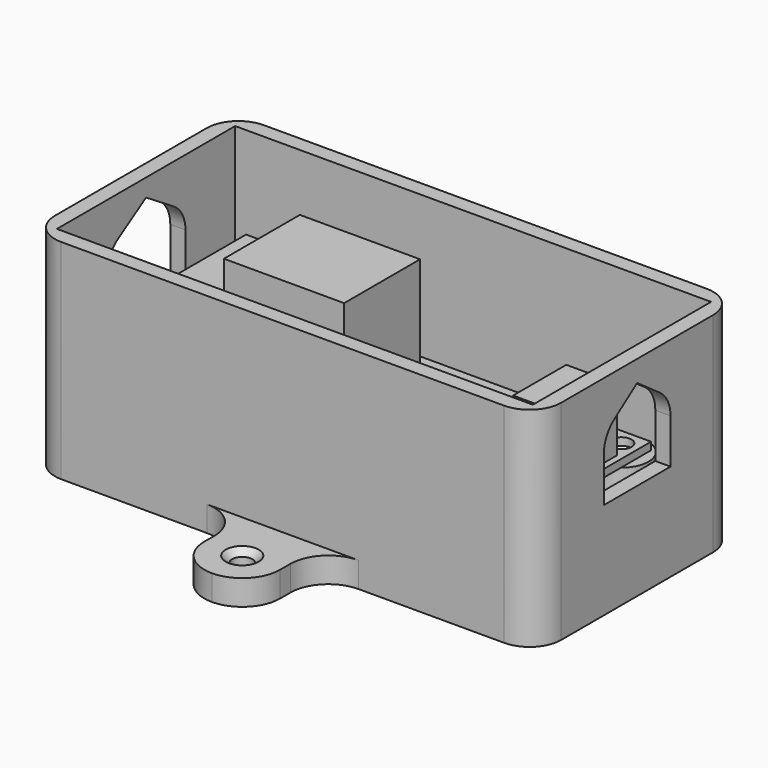
from build123d import *

# Parameters (mm, degrees)
F1_W          = 67.6
F1_H          = 21
F1_R          = 1.6
F2_DEPTH      = 1.2
F3_W          = 80
F3_H          = 40
F3_W_2        = 52
F3_H_2        = 28
F4_DEPTH      = 3
F5_R          = 4.25
F5_R_2        = 1.25
F6_DEPTH      = 14
F7_W          = 8
F7_H          = 15
F7_H_2        = 10.5
F8_DEPTH      = 10
F9_W          = 19
F9_H          = 15
F10_DEPTH     = 15.5
F11_W         = 80
F11_H         = 40
F11_W_2       = 75.2
F11_H_2       = 35.2
F12_DEPTH     = 30
F14_DEPTH     = 2.4
F16_DEPTH     = 2.4
F17_R         = 5
F18_W         = 12
F18_H         = 14
F18_R         = 1.6
F19_DEPTH     = 4
F20_R         = 5.99999
F21_R         = 2
F22_DEPTH     = 3
F23_S5_R      = 1.25
F23_T6_DEPTH  = 4
F23_S11_R     = 1.25
F23_T12_DEPTH = 4
F23_S17_R     = 1.25
F23_T18_DEPTH = 4
F23_S23_R     = 1.25
F23_T24_DEPTH = 4


# Not quite as in the source:
# - a fillet or chamfer that OpenCascade refuses, or shapes differently, is made with other operations: its cross-section is extruded or revolved along the edge and cut away or added
# - a fillet or chamfer is up to 0.001 mm smaller than in the source, because OpenCascade refuses the exact size


with BuildPart() as f2:
    # F1 (on Top) → F2 (new body)
    with BuildSketch(Plane.XY):
        Rectangle(F1_W, F1_H)
        with Locations((-31.2, -7.9)):
            Circle(F1_R, mode=Mode.SUBTRACT)
        with Locations((31.2, -7.9)):
            Circle(F1_R, mode=Mode.SUBTRACT)
        with Locations((-31.2, 7.9)):
            Circle(F1_R, mode=Mode.SUBTRACT)
        with Locations((31.2, 7.9)):
            Circle(F1_R, mode=Mode.SUBTRACT)
    extrude(amount=F2_DEPTH)

    # F7 (on face) → F8 (join)
    with BuildSketch(Plane.XY.offset(1.2)):
        with Locations((-23.8, 0)):
            Rectangle(F7_W, F7_H)
        with Locations((28.8, -0.25)):
            Rectangle(F7_W, F7_H_2)
    extrude(amount=F8_DEPTH)

    # F9 (on face) → F10 (join)
    with BuildSketch(Plane.XY.offset(1.2)):
        with Locations((-9.8, 0)):
            Rectangle(F9_W, F9_H)
    extrude(amount=F10_DEPTH)


with BuildPart() as f4:
    # F3 (on offset) → F4 (new body)
    with BuildSketch(Plane.XY.offset(-14)):
        Rectangle(F3_W, F3_H)
        Rectangle(F3_W_2, F3_H_2, mode=Mode.SUBTRACT)
    extrude(amount=F4_DEPTH)

    # F5 (on face) → F6 (join)
    with BuildSketch(Plane(origin=(0, 0, 0), x_dir=(1, 0, 0), z_dir=(0, 0, -1))):
        with Locations((-31.2, 7.9)):
            Circle(F5_R)
        with Locations((-31.2, 7.9)):
            Circle(F5_R_2, mode=Mode.SUBTRACT)
        with Locations((-31.2, -7.9)):
            Circle(F5_R)
        with Locations((-31.2, -7.9)):
            Circle(F5_R_2, mode=Mode.SUBTRACT)
        with Locations((31.2, 7.9)):
            Circle(F5_R)
        with Locations((31.2, 7.9)):
            Circle(F5_R_2, mode=Mode.SUBTRACT)
        with Locations((31.2, -7.9)):
            Circle(F5_R)
        with Locations((31.2, -7.9)):
            Circle(F5_R_2, mode=Mode.SUBTRACT)
    extrude(amount=F6_DEPTH)

    # F11 (on face) → F12 (join)
    with BuildSketch(Plane.XY.offset(-11)):
        Rectangle(F11_W, F11_H)
        Rectangle(F11_W_2, F11_H_2, mode=Mode.SUBTRACT)
    extrude(amount=F12_DEPTH)

    # F13 (on face) → F14 (cut, through all)
    with BuildSketch(Plane(origin=(-40, 0, 0), x_dir=(0, -1, 0), z_dir=(-1, 0, 0))):
        Polygon((-7.7893198468, 1.2333787745), (7.7893198468, 1.2333787745), (7.7893198468, 11.285850429), (0, 16.2070188671), (-7.7893198468, 11.285850429), align=None)
    extrude(amount=-F14_DEPTH, mode=Mode.SUBTRACT)

    # F15 (on face) → F16 (cut, through all)
    with BuildSketch(Plane.YZ.offset(40)):
        Polygon((-6.5914890729, 1.3349470682), (6.5914890729, 1.3349470682), (6.5914890729, 10.980901774), (0, 15.648432076), (-6.5914890729, 10.980901774), align=None)
    extrude(amount=-F16_DEPTH, mode=Mode.SUBTRACT)

    # F17
    f17_edges = [f4.edges().sort_by_distance(p)[0] for p in [
        (38.8, 6.591489, 10.980902),
        (-38.8, -7.78932, 11.28585),
        (-38.8, 7.78932, 11.28585),
        (38.8, -6.591489, 10.980902),
        (40, -20, 2.5),
        (40, 20, 2.5),
        (-40, 20, 2.5),
        (-40, -20, 2.5),
    ]]
    fillet(f17_edges, radius=F17_R)

    # F18 (on face) → F19 (join)
    with BuildSketch(Plane(origin=(0, 0, -14), x_dir=(1, 0, 0), z_dir=(0, 0, -1))):
        with Locations((0, 27)):
            Rectangle(F18_W, F18_H)
        with Locations((0, 28)):
            Circle(F18_R, mode=Mode.SUBTRACT)
        with Locations((-0.1473658485, -27)):
            Rectangle(F18_W, F18_H)
        with Locations((-0.1473658485, -28)):
            Circle(F18_R, mode=Mode.SUBTRACT)
    extrude(amount=-F19_DEPTH)

    # F20 (radius 6 in the source; OpenCascade refuses exactly that, so slightly less here)
    f20_edges = [f4.edges().sort_by_distance(p)[0] for p in [
        (6, -34, -12),
        (-6, -34, -12),
        (5.852634, 34, -12),
        (-6.147366, 34, -12),
        (5.852634, 20, -12),
        (-6.147366, 20, -12),
        (6, -20, -12),
        (-6, -20, -12),
    ]]
    fillet(f20_edges, radius=F20_R)

    # F21 (on face) → F22 (cut)
    with BuildSketch(Plane(origin=(0, 0, -14), x_dir=(1, 0, 0), z_dir=(0, 0, -1))):
        with Locations((-31.2, -7.9)):
            Circle(F21_R)
        with Locations((-31.2, 7.9)):
            Circle(F21_R)
        with Locations((31.2, -7.9)):
            Circle(F21_R)
        with Locations((31.2, 7.9)):
            Circle(F21_R)
    extrude(amount=-F22_DEPTH, mode=Mode.SUBTRACT)

    # F23: chamfer of 1 on 10 edges, made by hand


with BuildPart() as f23_tool2:
    # F23_s3 → F23_t4 (revolve)
    with BuildSketch(Plane.XZ.offset(-7.9)):
        Polygon((32.2, -11), (33.2, -12), (33.2, -11), align=None)
    revolve(axis=Axis((31.2, 7.9, -11), (0, 0, -1)))

    # F23_s5 → F23_t6 (cut, symmetric)
    with BuildSketch(Plane.XY.offset(-11.5)):
        with Locations((31.2, 7.9)):
            Circle(F23_S5_R)
    extrude(amount=F23_T6_DEPTH, both=True, mode=Mode.SUBTRACT)


with BuildPart() as f4_1:
    add(f4.part)

    # F23_t1: union F23_tool2
    add(f23_tool2.part)


with BuildPart() as f23_tool8:
    # F23_s9 → F23_t10 (revolve)
    with BuildSketch(Plane.XZ.offset(7.9)):
        Polygon((32.2, -11), (33.2, -12), (33.2, -11), align=None)
    revolve(axis=Axis((31.2, -7.9, -11), (0, 0, -1)))

    # F23_s11 → F23_t12 (cut, symmetric)
    with BuildSketch(Plane.XY.offset(-11.5)):
        with Locations((31.2, -7.9)):
            Circle(F23_S11_R)
    extrude(amount=F23_T12_DEPTH, both=True, mode=Mode.SUBTRACT)


with BuildPart() as f4_2:
    add(f4_1.part)

    # F23_t7: union F23_tool8
    add(f23_tool8.part)


with BuildPart() as f23_tool14:
    # F23_s15 → F23_t16 (revolve)
    with BuildSketch(Plane.XZ.offset(7.9)):
        Polygon((-30.2, -11), (-29.2, -12), (-29.2, -11), align=None)
    revolve(axis=Axis((-31.2, -7.9, -11), (0, 0, -1)))

    # F23_s17 → F23_t18 (cut, symmetric)
    with BuildSketch(Plane.XY.offset(-11.5)):
        with Locations((-31.2, -7.9)):
            Circle(F23_S17_R)
    extrude(amount=F23_T18_DEPTH, both=True, mode=Mode.SUBTRACT)


with BuildPart() as f4_3:
    add(f4_2.part)

    # F23_t13: union F23_tool14
    add(f23_tool14.part)


with BuildPart() as f23_tool20:
    # F23_s21 → F23_t22 (revolve)
    with BuildSketch(Plane.XZ.offset(-7.9)):
        Polygon((-30.2, -11), (-29.2, -12), (-29.2, -11), align=None)
    revolve(axis=Axis((-31.2, 7.9, -11), (0, 0, -1)))

    # F23_s23 → F23_t24 (cut, symmetric)
    with BuildSketch(Plane.XY.offset(-11.5)):
        with Locations((-31.2, 7.9)):
            Circle(F23_S23_R)
    extrude(amount=F23_T24_DEPTH, both=True, mode=Mode.SUBTRACT)


with BuildPart() as f4_4:
    add(f4_3.part)

    # F23_t19: union F23_tool20
    add(f23_tool20.part)

    # F23_s25 → F23_t26 (revolve, cut)
    with BuildSketch(Plane.XZ.offset(7.9)):
        Polygon((-29.95, -1), (-28.95, 0), (-29.95, 0), align=None)
    revolve(axis=Axis((-31.2, -7.9, 0), (0, 0, -1)), mode=Mode.SUBTRACT)

    # F23_s27 → F23_t28 (revolve, cut)
    with BuildSketch(Plane.XZ.offset(-7.9)):
        Polygon((-28.95, 0), (-29.95, -1), (-29.95, 0), align=None)
    revolve(axis=Axis((-31.2, 7.9, 0), (0, 0, -1)), mode=Mode.SUBTRACT)

    # F23_s29 → F23_t30 (revolve, cut)
    with BuildSketch(Plane.XZ.offset(7.9)):
        Polygon((33.45, 0), (32.45, -1), (32.45, 0), align=None)
    revolve(axis=Axis((31.2, -7.9, 0), (0, 0, -1)), mode=Mode.SUBTRACT)

    # F23_s31 → F23_t32 (revolve, cut)
    with BuildSketch(Plane.XZ.offset(-7.9)):
        Polygon((33.45, 0), (32.45, -1), (32.45, 0), align=None)
    revolve(axis=Axis((31.2, 7.9, 0), (0, 0, -1)), mode=Mode.SUBTRACT)

    # F23_s33 → F23_t34 (revolve, cut)
    with BuildSketch(Plane.XZ.offset(28)):
        Polygon((1.6, -11), (2.6, -10), (1.6, -10), align=None)
    revolve(axis=Axis((0, -28, -10), (0, 0, -1)), mode=Mode.SUBTRACT)

    # F23_s35 → F23_t36 (revolve, cut)
    with BuildSketch(Plane.XZ.offset(-28)):
        Polygon((2.4526341515, -10), (1.4526341515, -11), (1.4526341515, -10), align=None)
    revolve(axis=Axis((-0.1473658485, 28, -10), (0, 0, -1)), mode=Mode.SUBTRACT)


solid = Compound([f2.part, f4_4.part])
